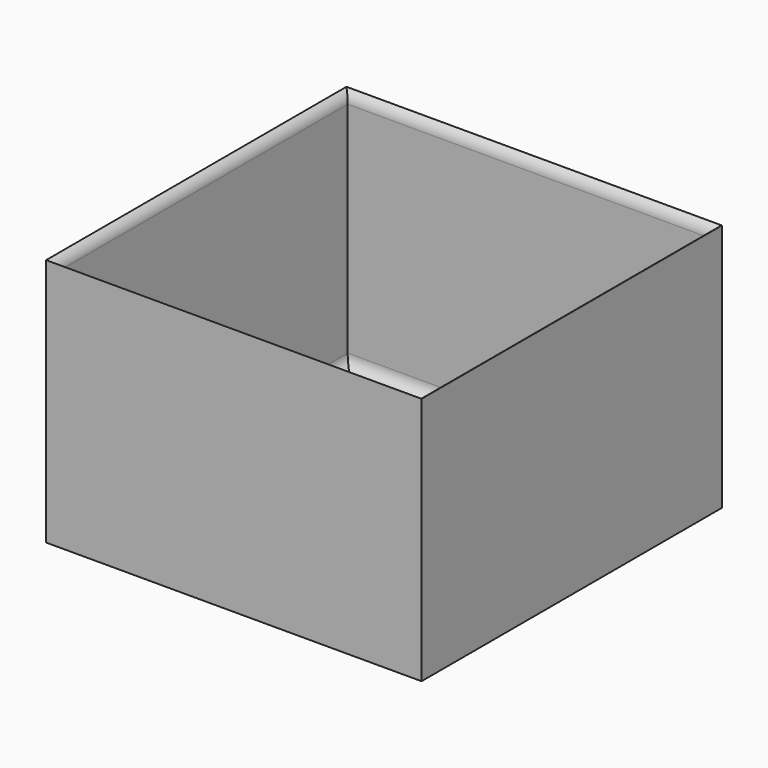
from build123d import *

# Parameters (mm, degrees)
F0_W         = 152.4
F0_H         = 101.6
F1_DEPTH     = 152.4
F2_T         = -2.54
F3_T1_DEPTH  = 147.32
F3_T3_DEPTH  = 147.32
F3_T5_DEPTH  = 147.32
F3_T7_DEPTH  = 147.32
F3_T13_DEPTH = 160.02
F3_T19_DEPTH = 160.02
F3_T28_DEPTH = 160.02
F3_T34_DEPTH = 160.02
F3_T43_DEPTH = 160.02
F3_T49_DEPTH = 160.02
F3_T58_DEPTH = 160.02
F3_T64_DEPTH = 160.02


# Not quite as in the source:
# - a fillet or chamfer that OpenCascade refuses, or shapes differently, is made with other operations: its cross-section is extruded or revolved along the edge and cut away or added


with BuildPart() as f1:
    # F0 (on Front) → F1 (new body)
    with BuildSketch(Plane.XZ):
        with Locations((-25.9277992306, 50.8)):
            Rectangle(F0_W, F0_H)
    extrude(amount=F1_DEPTH)

    # F2
    f2_openings = [f1.faces().sort_by_distance(p)[0] for p in [
        (-25.927799, -76.2, 101.6),
    ]]
    offset(amount=F2_T, openings=f2_openings)

    # F3: fillet of radius 5.08 on 8 edges, made by hand

    # F3_s2 → F3_t1 (join)
    with BuildSketch(Plane.XZ.offset(2.54)):
        with BuildLine():
            ThreePointArc((47.7322007694, 7.62), (46.2443032178, 4.0278975516), (42.6522007694, 2.54))
            Line((42.6522007694, 2.54), (47.7322007694, 2.54))
            Line((47.7322007694, 2.54), (47.7322007694, 7.62))
        make_face()
        with BuildLine():
            ThreePointArc((-99.5877992306, 7.62), (-98.0999016791, 4.0278975516), (-94.5077992306, 2.54))
            Line((-94.5077992306, 2.54), (-99.5877992306, 2.54))
            Line((-99.5877992306, 2.54), (-99.5877992306, 7.62))
        make_face()
    extrude(amount=F3_T1_DEPTH)

    # F3_s4 → F3_t3 (join)
    with BuildSketch(Plane.YZ.offset(-99.5877992306)):
        with BuildLine():
            ThreePointArc((-2.54, 7.62), (-4.0278975516, 4.0278975516), (-7.62, 2.54))
            Line((-7.62, 2.54), (-2.54, 2.54))
            Line((-2.54, 2.54), (-2.54, 7.62))
        make_face()
        with BuildLine():
            ThreePointArc((-149.86, 7.62), (-148.3721024484, 4.0278975516), (-144.78, 2.54))
            Line((-144.78, 2.54), (-149.86, 2.54))
            Line((-149.86, 2.54), (-149.86, 7.62))
        make_face()
    extrude(amount=F3_T3_DEPTH)

    # F3_s6 → F3_t5 (cut)
    with BuildSketch(Plane.YZ.offset(-99.5877992306)):
        with BuildLine():
            ThreePointArc((2.54, 101.6), (-1.0521024484, 100.1121024484), (-2.54, 96.52))
            Line((-2.54, 96.52), (-2.54, 101.6))
            Line((-2.54, 101.6), (2.54, 101.6))
        make_face()
        with BuildLine():
            ThreePointArc((-154.94, 101.6), (-151.3478975516, 100.1121024484), (-149.86, 96.52))
            Line((-149.86, 96.52), (-149.86, 101.6))
            Line((-149.86, 101.6), (-154.94, 101.6))
        make_face()
    extrude(amount=F3_T5_DEPTH, mode=Mode.SUBTRACT)

    # F3_s8 → F3_t7 (cut)
    with BuildSketch(Plane.XZ.offset(2.54)):
        with BuildLine():
            ThreePointArc((52.8122007694, 101.6), (49.2200983209, 100.1121024484), (47.7322007694, 96.52))
            Line((47.7322007694, 96.52), (47.7322007694, 101.6))
            Line((47.7322007694, 101.6), (52.8122007694, 101.6))
        make_face()
        with BuildLine():
            ThreePointArc((-104.6677992306, 101.6), (-101.0756967822, 100.1121024484), (-99.5877992306, 96.52))
            Line((-99.5877992306, 96.52), (-99.5877992306, 101.6))
            Line((-99.5877992306, 101.6), (-104.6677992306, 101.6))
        make_face()
    extrude(amount=F3_T7_DEPTH, mode=Mode.SUBTRACT)


with BuildPart() as f3_tool11:
    # F3_s12 → F3_t13 (new body)
    with BuildSketch(Plane.XZ.offset(-10.16)):
        with BuildLine():
            ThreePointArc((52.8122007694, 101.6), (49.2200983209, 100.1121024484), (47.7322007694, 96.52))
            Line((47.7322007694, 96.52), (47.7322007694, 101.6))
            Line((47.7322007694, 101.6), (52.8122007694, 101.6))
        make_face()
    extrude(amount=F3_T13_DEPTH)

    split(bisect_by=Plane.XZ, keep=Keep.TOP)

    split(bisect_by=Plane.YZ.offset(50.2722007694), keep=Keep.BOTTOM)

    split(bisect_by=Plane.XZ.offset(2.54), keep=Keep.BOTTOM)


with BuildPart() as f3_tool17:
    # F3_s18 → F3_t19 (new body)
    with BuildSketch(Plane.YZ.offset(60.4322007694)):
        with BuildLine():
            ThreePointArc((2.54, 101.6), (-1.0521024484, 100.1121024484), (-2.54, 96.52))
            Line((-2.54, 96.52), (-2.54, 101.6))
            Line((-2.54, 101.6), (2.54, 101.6))
        make_face()
    extrude(amount=-F3_T19_DEPTH)

    split(bisect_by=Plane.XZ, keep=Keep.TOP)

    split(bisect_by=Plane.YZ.offset(50.2722007694), keep=Keep.BOTTOM)

    split(bisect_by=Plane.YZ.offset(47.7322007694), keep=Keep.TOP)


with BuildPart() as f3_tool11_1:
    add(f3_tool11.part)

    # F3_t23: intersect F3_tool17
    add(f3_tool17.part, mode=Mode.INTERSECT)


with BuildPart() as f1_1:
    add(f1.part)

    # F3_t9: cut F3_tool11
    add(f3_tool11_1.part, mode=Mode.SUBTRACT)


with BuildPart() as f3_tool26:
    # F3_s27 → F3_t28 (new body)
    with BuildSketch(Plane.YZ.offset(47.7322007694)):
        with BuildLine():
            ThreePointArc((2.54, 101.6), (-1.0521024484, 100.1121024484), (-2.54, 96.52))
            Line((-2.54, 96.52), (-2.54, 101.6))
            Line((-2.54, 101.6), (2.54, 101.6))
        make_face()
    extrude(amount=-F3_T28_DEPTH)

    split(bisect_by=Plane.YZ.offset(-102.1277992306), keep=Keep.TOP)

    split(bisect_by=Plane.XZ, keep=Keep.TOP)

    split(bisect_by=Plane.YZ.offset(-99.5877992306), keep=Keep.BOTTOM)


with BuildPart() as f3_tool32:
    # F3_s33 → F3_t34 (new body)
    with BuildSketch(Plane.XZ.offset(-10.16)):
        with BuildLine():
            ThreePointArc((-104.6677992306, 101.6), (-101.0756967822, 100.1121024484), (-99.5877992306, 96.52))
            Line((-99.5877992306, 96.52), (-99.5877992306, 101.6))
            Line((-99.5877992306, 101.6), (-104.6677992306, 101.6))
        make_face()
    extrude(amount=F3_T34_DEPTH)

    split(bisect_by=Plane.YZ.offset(-102.1277992306), keep=Keep.TOP)

    split(bisect_by=Plane.XZ, keep=Keep.TOP)

    split(bisect_by=Plane.XZ.offset(2.54), keep=Keep.BOTTOM)


with BuildPart() as f3_tool26_1:
    add(f3_tool26.part)

    # F3_t38: intersect F3_tool32
    add(f3_tool32.part, mode=Mode.INTERSECT)


with BuildPart() as f1_2:
    add(f1_1.part)

    # F3_t24: cut F3_tool26
    add(f3_tool26_1.part, mode=Mode.SUBTRACT)


with BuildPart() as f3_tool41:
    # F3_s42 → F3_t43 (new body)
    with BuildSketch(Plane.XZ.offset(2.54)):
        with BuildLine():
            ThreePointArc((52.8122007694, 101.6), (49.2200983209, 100.1121024484), (47.7322007694, 96.52))
            Line((47.7322007694, 96.52), (47.7322007694, 101.6))
            Line((47.7322007694, 101.6), (52.8122007694, 101.6))
        make_face()
    extrude(amount=F3_T43_DEPTH)

    split(bisect_by=Plane.XZ.offset(152.4), keep=Keep.BOTTOM)

    split(bisect_by=Plane.YZ.offset(50.2722007694), keep=Keep.BOTTOM)

    split(bisect_by=Plane.XZ.offset(149.86), keep=Keep.TOP)


with BuildPart() as f3_tool47:
    # F3_s48 → F3_t49 (new body)
    with BuildSketch(Plane.YZ.offset(60.4322007694)):
        with BuildLine():
            ThreePointArc((-154.94, 101.6), (-151.3478975516, 100.1121024484), (-149.86, 96.52))
            Line((-149.86, 96.52), (-149.86, 101.6))
            Line((-149.86, 101.6), (-154.94, 101.6))
        make_face()
    extrude(amount=-F3_T49_DEPTH)

    split(bisect_by=Plane.XZ.offset(152.4), keep=Keep.BOTTOM)

    split(bisect_by=Plane.YZ.offset(50.2722007694), keep=Keep.BOTTOM)

    split(bisect_by=Plane.YZ.offset(47.7322007694), keep=Keep.TOP)


with BuildPart() as f3_tool41_1:
    add(f3_tool41.part)

    # F3_t53: intersect F3_tool47
    add(f3_tool47.part, mode=Mode.INTERSECT)


with BuildPart() as f1_3:
    add(f1_2.part)

    # F3_t39: cut F3_tool41
    add(f3_tool41_1.part, mode=Mode.SUBTRACT)


with BuildPart() as f3_tool56:
    # F3_s57 → F3_t58 (new body)
    with BuildSketch(Plane.XZ.offset(2.54)):
        with BuildLine():
            ThreePointArc((-104.6677992306, 101.6), (-101.0756967822, 100.1121024484), (-99.5877992306, 96.52))
            Line((-99.5877992306, 96.52), (-99.5877992306, 101.6))
            Line((-99.5877992306, 101.6), (-104.6677992306, 101.6))
        make_face()
    extrude(amount=F3_T58_DEPTH)

    split(bisect_by=Plane.YZ.offset(-102.1277992306), keep=Keep.TOP)

    split(bisect_by=Plane.XZ.offset(152.4), keep=Keep.BOTTOM)

    split(bisect_by=Plane.XZ.offset(149.86), keep=Keep.TOP)


with BuildPart() as f3_tool62:
    # F3_s63 → F3_t64 (new body)
    with BuildSketch(Plane.YZ.offset(47.7322007694)):
        with BuildLine():
            ThreePointArc((-154.94, 101.6), (-151.3478975516, 100.1121024484), (-149.86, 96.52))
            Line((-149.86, 96.52), (-149.86, 101.6))
            Line((-149.86, 101.6), (-154.94, 101.6))
        make_face()
    extrude(amount=-F3_T64_DEPTH)

    split(bisect_by=Plane.YZ.offset(-102.1277992306), keep=Keep.TOP)

    split(bisect_by=Plane.XZ.offset(152.4), keep=Keep.BOTTOM)

    split(bisect_by=Plane.YZ.offset(-99.5877992306), keep=Keep.BOTTOM)


with BuildPart() as f3_tool56_1:
    add(f3_tool56.part)

    # F3_t68: intersect F3_tool62
    add(f3_tool62.part, mode=Mode.INTERSECT)


with BuildPart() as f1_4:
    add(f1_3.part)

    # F3_t54: cut F3_tool56
    add(f3_tool56_1.part, mode=Mode.SUBTRACT)


solid = f1_4.part
